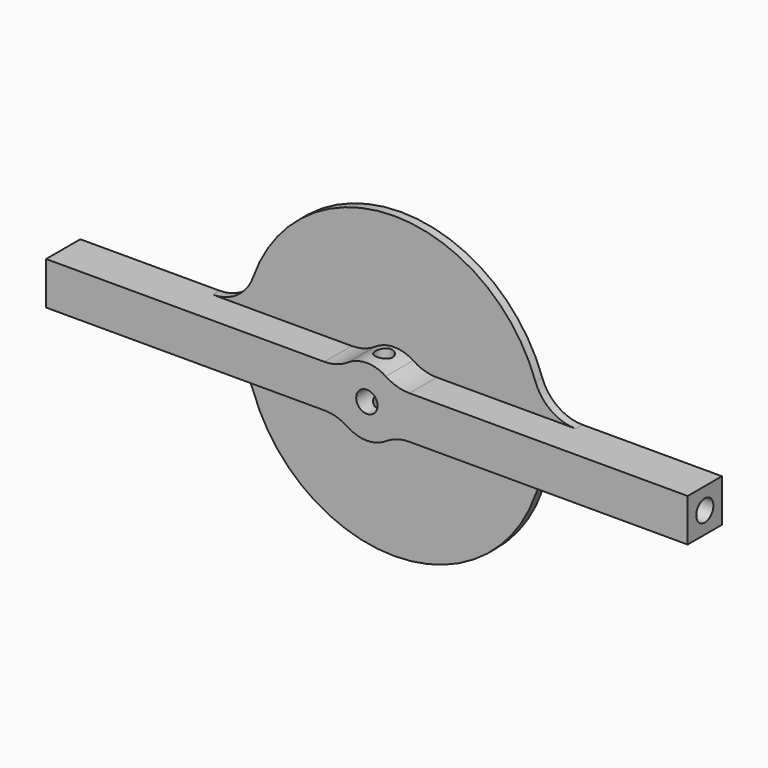
from build123d import *

# Parameters (mm, degrees)
F0_R          = 2.5
F1_DEPTH      = 10
F2_R          = 35
F2_R_2        = 2.5
F3_DEPTH      = 2
F4_R          = 2.5
F5_DEPTH      = 25
F6_R          = 2
F7_DEPTH      = 35.001
F7_DEPTH_BACK = 35.001
F8_R          = 10


# Not quite as in the source:
# - a pattern or mirror of a feature is missing from the dataset's text; its kind, count and spacing are read off the source's solid


with BuildPart() as f1:
    # F0 (on Front) → F1 (new body)
    with BuildSketch(Plane.XZ):
        with BuildLine():
            Line((75, 5), (6.2449979984, 5))
            ThreePointArc((6.2449979984, 5), (0, 8), (-6.2449979984, 5))
            Line((-6.2449979984, 5), (-75, 5))
            Line((-75, 5), (-75, -5))
            Line((-75, -5), (-6.2449979984, -5))
            ThreePointArc((-6.2449979984, -5), (0, -8), (6.2449979984, -5))
            Line((6.2449979984, -5), (75, -5))
            Line((75, -5), (75, 5))
        make_face()
        Circle(F0_R, mode=Mode.SUBTRACT)
    extrude(amount=F1_DEPTH)

    # F2 (on face) → F3 (join)
    with BuildSketch(Plane(origin=(0, 0, 0), x_dir=(-1, 0, 0), z_dir=(0, 1, 0))):
        Circle(F2_R)
        Circle(F2_R_2, mode=Mode.SUBTRACT)
    extrude(amount=-F3_DEPTH)

    # F4 (on face) → F5 (cut)
    with BuildSketch(Plane(origin=(-75, 0, 0), x_dir=(0, -1, 0), z_dir=(-1, 0, 0))):
        with Locations((5, 0)):
            Circle(F4_R)
    f5 = extrude(amount=-F5_DEPTH, mode=Mode.SUBTRACT)

    # F5_copies: F5 across plane
    add(f5.mirror(Plane(origin=(0, 0, 0), x_dir=(0, 0, 1), z_dir=(1, 0, 0))), mode=Mode.SUBTRACT)

    # F6 (on Top) → F7 (cut, two sides)
    with BuildSketch(Plane.XY) as f7_sk:
        with Locations((0, -5)):
            Circle(F6_R)
    extrude(amount=-F7_DEPTH, mode=Mode.SUBTRACT)
    extrude(f7_sk.sketch, amount=F7_DEPTH_BACK, mode=Mode.SUBTRACT)

    # F8
    f8_edges = [f1.edges().sort_by_distance(p)[0] for p in [
        (-6.244998, -6, 5),
        (6.244998, -6, 5),
        (6.244998, -6, -5),
        (-6.244998, -6, -5),
        (34.641016, -1, 5),
        (34.641016, -1, -5),
        (-34.641016, -1, -5),
        (-34.641016, -1, 5),
    ]]
    fillet(f8_edges, radius=F8_R)


solid = f1.part
